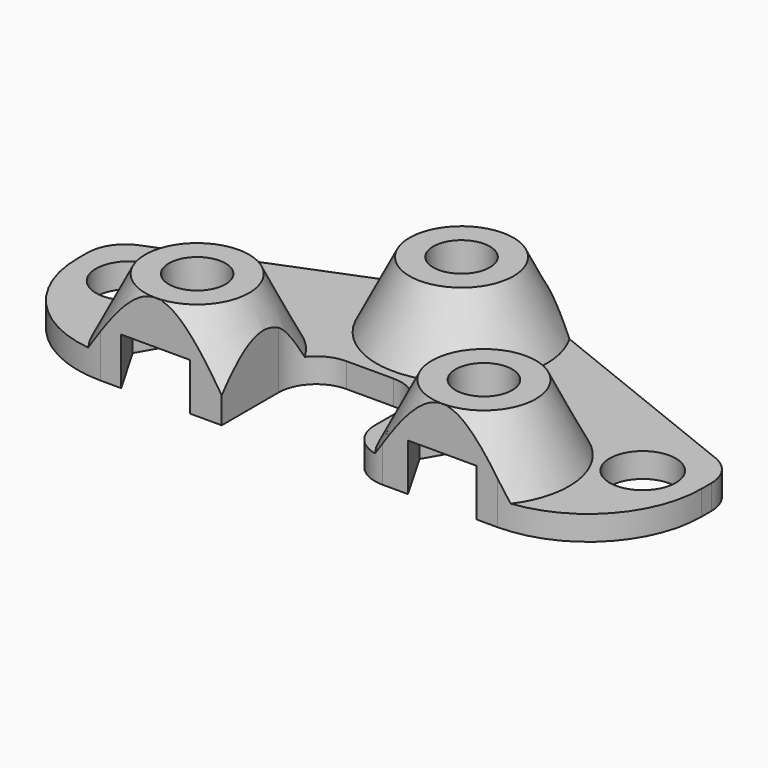
from build123d import *

# Parameters (mm, degrees)
F0_W         = 33
F0_H         = 14
F0_R         = 1.75
F1_DEPTH     = 4.8
F2_R         = 1.5
F4_DEPTH     = 4.8
F2_W         = 33
F2_H         = 14
F2_R_2       = 2.5
F2_R_3       = 1.75
F5_DEPTH     = 3.5
F7_DEPTH     = 2.5
F8_W         = 6.5
F8_H         = 5.7518341467
F9_DEPTH     = 12.5
F10_R        = 6
F11_T1_DEPTH = 79.0934091739
F12_R        = 2


# Not quite as in the source:
# - a fillet or chamfer that OpenCascade refuses, or shapes differently, is made with other operations: its cross-section is extruded or revolved along the edge and cut away or added


with BuildPart() as f1:
    # F0 (on Top) → F1 (new body)
    with BuildSketch(Plane.XY):
        with Locations((0, 1.2481658533)):
            Rectangle(F0_W, F0_H)
        with Locations((-13.585, 0)):
            Circle(F0_R, mode=Mode.SUBTRACT)
        with Locations((13.585, 0)):
            Circle(F0_R, mode=Mode.SUBTRACT)
    extrude(amount=F1_DEPTH)

    # F2 (on face) → F4 (cut, through all)
    with BuildSketch(Plane.XY.offset(4.8)):
        with Locations((-7.585, -3)):
            Circle(F2_R)
        with Locations((0, 5)):
            Circle(F2_R)
        with Locations((7.585, -3)):
            Circle(F2_R)
    extrude(amount=-F4_DEPTH, mode=Mode.SUBTRACT)

    # F2 (on face) → F5 (cut)
    with BuildSketch(Plane.XY.offset(4.8)):
        with Locations((0, 1.2481658533)):
            Rectangle(F2_W, F2_H)
        with Locations((-7.585, -3)):
            Circle(F2_R_2, mode=Mode.SUBTRACT)
        with Locations((-13.585, 0)):
            Circle(F2_R_3, mode=Mode.SUBTRACT)
        with Locations((7.585, -3)):
            Circle(F2_R_2, mode=Mode.SUBTRACT)
        with Locations((13.585, 0)):
            Circle(F2_R_3, mode=Mode.SUBTRACT)
        with Locations((0, 5)):
            Circle(F2_R_2, mode=Mode.SUBTRACT)
    extrude(amount=-F5_DEPTH, mode=Mode.SUBTRACT)

    # F6: chamfer of 4 x 2 on 3 edges, made by hand


with BuildPart() as f6_tool2:
    # F6_s3 → F6_t4 (revolve)
    with BuildSketch(Plane.XZ.offset(3)):
        Polygon((-3.085, 1.3), (-5.085, 5.3), (-5.085, 1.3), align=None)
    revolve(axis=Axis((-7.585, -3, 1.3), (0, 0, 1)))

    split(bisect_by=Plane.XZ.offset(5.7518341467), keep=Keep.BOTTOM)

    split(bisect_by=Plane.XY.offset(4.8), keep=Keep.BOTTOM)


with BuildPart() as f1_1:
    add(f1.part)

    # F6_t1: union F6_tool2
    add(f6_tool2.part)


with BuildPart() as f6_tool8:
    # F6_s9 → F6_t10 (revolve)
    with BuildSketch(Plane.XZ.offset(-5)):
        Polygon((4.5, 1.3), (2.5, 5.3), (2.5, 1.3), align=None)
    revolve(axis=Axis((0, 5, 1.3), (0, 0, 1)))

    split(bisect_by=Plane.XZ.offset(-8.2481658533), keep=Keep.TOP)

    split(bisect_by=Plane.XY.offset(4.8), keep=Keep.BOTTOM)


with BuildPart() as f1_2:
    add(f1_1.part)

    # F6_t7: union F6_tool8
    add(f6_tool8.part)


with BuildPart() as f6_tool14:
    # F6_s15 → F6_t16 (revolve)
    with BuildSketch(Plane.XZ.offset(3)):
        Polygon((12.085, 1.3), (10.085, 5.3), (10.085, 1.3), align=None)
    revolve(axis=Axis((7.585, -3, 1.3), (0, 0, 1)))

    split(bisect_by=Plane.XZ.offset(5.7518341467), keep=Keep.BOTTOM)

    split(bisect_by=Plane.XY.offset(4.8), keep=Keep.BOTTOM)


with BuildPart() as f1_3:
    add(f1_2.part)

    # F6_t13: union F6_tool14
    add(f6_tool14.part)

    # F3 (on face) → F7 (cut)
    with BuildSketch(Plane(origin=(0, 0, 0), x_dir=(1, 0, 0), z_dir=(0, 0, -1))):
        Polygon((-5.8818167059, 5.95), (-9.2881832941, 5.95), (-9.4025944029, 5.7518341467), (-5.7674055971, 5.7518341467), align=None)
        Polygon((9.4025944029, 5.7518341467), (5.7674055971, 5.7518341467), (4.1786334118, 3), (5.8818167059, 0.05), (9.2881832941, 0.05), (10.9913665882, 3), align=None)
        Polygon((-1.7031832941, -7.95), (1.7031832941, -7.95), (3.4063665882, -5), (1.7031832941, -2.05), (-1.7031832941, -2.05), (-3.4063665882, -5), align=None)
        Polygon((-5.7674055971, 5.7518341467), (-9.4025944029, 5.7518341467), (-10.9913665882, 3), (-9.2881832941, 0.05), (-5.8818167059, 0.05), (-4.1786334118, 3), align=None)
    extrude(amount=-F7_DEPTH, mode=Mode.SUBTRACT)

    # F8 (on face) → F9 (cut, symmetric)
    with BuildSketch(Plane.XY.offset(1.3)):
        with Locations((-0.835, -2.8759170733)):
            Rectangle(F8_W, F8_H)
    extrude(amount=F9_DEPTH, both=True, mode=Mode.SUBTRACT)

    # F10
    f10_edges = [f1_3.edges().sort_by_distance(p)[0] for p in [
        (-16.5, -5.751834, 0.65),
        (16.5, -5.751834, 0.65),
    ]]
    fillet(f10_edges, radius=F10_R)

    # F11: chamfer of 6 x 15 on 2 edges, made by hand

    # F11_s2 → F11_t1 (cut)
    with BuildSketch(Plane.XY.offset(-38.896704587)):
        Polygon((-1.5, 8.2481658533), (-16.5, 2.2481658533), (-16.5, 8.2481658533), align=None)
        Polygon((16.5, 2.2481658533), (1.5, 8.2481658533), (16.5, 8.2481658533), align=None)
    extrude(amount=F11_T1_DEPTH, mode=Mode.SUBTRACT)

    # F12 (call 1 of 5: OpenCascade refuses the feature's edges together)
    f12_edges = [f1_3.edges().sort_by_distance(p)[0] for p in [
        (-4.085, 0, 0.65),
    ]]
    fillet(f12_edges, radius=F12_R)

    # F12#2 (call 2 of 5)
    f12_2_edges = [f1_3.edges().sort_by_distance(p)[0] for p in [
        (2.415, 0, 0.65),
    ]]
    fillet(f12_2_edges, radius=F12_R)

    # F12#3 (call 3 of 5)
    f12_3_edges = [f1_3.edges().sort_by_distance(p)[0] for p in [
        (2.415, -5.751834, 0.65),
    ]]
    fillet(f12_3_edges, radius=F12_R)

    # F12#4 (call 4 of 5)
    f12_4_edges = [f1_3.edges().sort_by_distance(p)[0] for p in [
        (16.5, 2.248166, 0.65),
    ]]
    fillet(f12_4_edges, radius=F12_R)

    # F12#5 (call 5 of 5)
    f12_5_edges = [f1_3.edges().sort_by_distance(p)[0] for p in [
        (-16.5, 2.248166, 0.65),
    ]]
    fillet(f12_5_edges, radius=F12_R)


solid = f1_3.part
